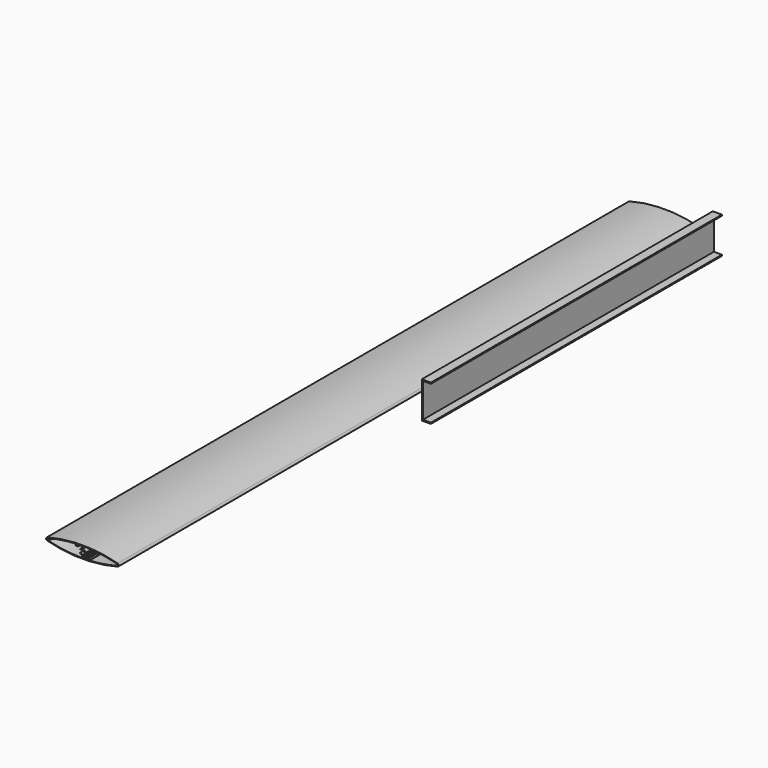
from build123d import *

# Parameters (mm, degrees)
F1_DEPTH = 2000
F3_DEPTH = 1000


# Not quite as in the source:
# - ends of sketch curves that miss each other by under 0.0002 mm in the source are joined


with BuildPart() as f1:
    # F0 (on Front) → F1 (new body)
    with BuildSketch(Plane.XZ):
        with BuildLine():
            ThreePointArc((-17.5657668552, -7.9557874553), (-114.482143, 4.708559), (-211.3985191448, -7.9557874553))
            ThreePointArc((-211.3985191468, -7.9557874481), (-214.482143, -11.966441), (-211.3985191468, -15.9770945519))
            ThreePointArc((-211.3985191448, -15.9770945447), (-114.482143, -28.641441), (-17.5657668552, -15.9770945447))
            ThreePointArc((-17.5657668532, -15.9770945519), (-14.482143, -11.966441), (-17.5657668532, -7.9557874481))
        make_face()
        with BuildLine():
            ThreePointArc((-208.9077742877, -13.5769296747), (-212.482143, -11.966441), (-208.9077742877, -10.3559523253))
            ThreePointArc((-208.9077742877, -10.3559523253), (-207.7533400412, -10.4775188222), (-207.2617892935, -9.425913054))
            ThreePointArc((-207.2617892935, -9.425913054), (-207.1910048941, -9.0656220914), (-206.8932051271, -8.8508305))
            ThreePointArc((-206.8932051271, -8.8508305), (-170.9950203177, -1.5722317693), (-134.5581469899, 2.1710198123))
            ThreePointArc((-134.5581469899, 2.1710198123), (-133.7402264674, 1.8171851888), (-133.5293940092, 0.9513082288))
            ThreePointArc((-133.5293940092, 0.9513082288), (-133.5025335267, -0.9954988279), (-132.5907607495, -2.7158037784))
            ThreePointArc((-132.5907607495, -2.7158037784), (-131.1791989669, -2.8023715374), (-131.0926316821, -1.3908097188))
            ThreePointArc((-131.0926316821, -1.3908097188), (-129.482143, 2.183559), (-127.8716543253, -1.3908097123))
            ThreePointArc((-127.8716543253, -1.3908097123), (-127.7850870331, -2.8023715374), (-126.3735252432, -2.7158037849))
            ThreePointArc((-126.3735252432, -2.7158037849), (-125.4236024617, -0.8328985575), (-125.5217918168, 1.2737680574))
            ThreePointArc((-125.5217918168, 1.2737680574), (-125.3812649978, 2.1537940521), (-124.5944440182, 2.5722506744))
            ThreePointArc((-124.5944440182, 2.5722506744), (-120.5413197711, 2.6596262173), (-116.4874880026, 2.7031994831))
            ThreePointArc((-116.4874880026, 2.7031994831), (-115.776928495, 2.412208007), (-115.482143, 1.703214))
            Line((-115.482143, 1.703214), (-115.482143, -2.986463))
            ThreePointArc((-115.482143, -2.986463), (-115.7019536269, -3.6120063974), (-116.2647520841, -3.9625476222))
            ThreePointArc((-116.2647520841, -3.9625476222), (-118.8659014588, -5.03660249), (-120.9507289205, -6.926858062))
            ThreePointArc((-120.9507289205, -6.926858062), (-120.7764600793, -8.3302931018), (-119.3730248982, -8.1560240793))
            ThreePointArc((-119.3730248982, -8.1560240793), (-108.282143, -11.966441), (-119.3730247168, -15.7768577794))
            ThreePointArc((-119.3730247168, -15.7768577794), (-120.7764600793, -15.6025888982), (-120.9507291018, -17.0060240793))
            ThreePointArc((-120.9507291018, -17.0060240793), (-118.8659014588, -18.89627951), (-116.2647520265, -19.9703341189))
            ThreePointArc((-116.2647520265, -19.9703341189), (-115.7019536269, -20.3208756026), (-115.482143, -20.946419))
            Line((-115.482143, -20.946419), (-115.482143, -25.636096))
            ThreePointArc((-115.482143, -25.636096), (-115.776928495, -26.345090007), (-116.4874880038, -26.6360817154))
            ThreePointArc((-116.4874880038, -26.6360817154), (-162.0425086737, -23.6145958983), (-206.8932050038, -15.0820510151))
            ThreePointArc((-206.8932050038, -15.0820510151), (-207.1910048941, -14.8672599086), (-207.2617897315, -14.5069688654))
            ThreePointArc((-207.2617897315, -14.5069688654), (-207.7533400412, -13.4553631778), (-208.9077742877, -13.5769296747))
        make_face(mode=Mode.SUBTRACT)
        with BuildLine():
            ThreePointArc((-112.6995339159, -3.9625476222), (-113.2623323731, -3.6120063974), (-113.482143, -2.986463))
            Line((-113.482143, -2.986463), (-113.482143, 1.703214))
            ThreePointArc((-113.482143, 1.703214), (-113.187357505, 2.412208007), (-112.4767979962, 2.7031997154))
            ThreePointArc((-112.4767979962, 2.7031997154), (-66.9217773263, -0.3182861017), (-22.0710809962, -8.8508309849))
            ThreePointArc((-22.0710809962, -8.8508309849), (-21.7732811059, -9.0656220914), (-21.7024962685, -9.4259131346))
            ThreePointArc((-21.7024962685, -9.4259131346), (-21.2109459588, -10.4775188222), (-20.0565117188, -10.3559523179))
            ThreePointArc((-20.0565117188, -10.3559523179), (-16.482143, -11.966441), (-20.0565117123, -13.5769296747))
            ThreePointArc((-20.0565117123, -13.5769296747), (-21.2109459588, -13.4553631778), (-21.7024967065, -14.506968946))
            ThreePointArc((-21.7024967065, -14.506968946), (-21.7732811059, -14.8672599086), (-22.0710808729, -15.0820515))
            ThreePointArc((-22.0710808729, -15.0820515), (-57.9692656823, -22.3606502307), (-94.4061390101, -26.1039018123))
            ThreePointArc((-94.4061390101, -26.1039018123), (-95.2240595326, -25.7500671888), (-95.4348919908, -24.8841902288))
            ThreePointArc((-95.4348919908, -24.8841902288), (-95.4617524733, -22.9373831721), (-96.3735252505, -21.2170782216))
            ThreePointArc((-96.3735252505, -21.2170782216), (-97.7850870331, -21.1305104626), (-97.8716543179, -22.5420722812))
            ThreePointArc((-97.8716543179, -22.5420722812), (-99.482143, -26.116441), (-101.0926316747, -22.5420722877))
            ThreePointArc((-101.0926316747, -22.5420722877), (-101.1791989669, -21.1305104626), (-102.5907607568, -21.2170782151))
            ThreePointArc((-102.5907607568, -21.2170782151), (-103.5406835383, -23.0999834425), (-103.4424941832, -25.2066500574))
            ThreePointArc((-103.4424941832, -25.2066500574), (-103.5830210022, -26.0866760521), (-104.3698419818, -26.5051326744))
            ThreePointArc((-104.3698419818, -26.5051326744), (-108.4229662289, -26.5925082173), (-112.4767979974, -26.6360814831))
            ThreePointArc((-112.4767979974, -26.6360814831), (-113.187357505, -26.345090007), (-113.482143, -25.636096))
            Line((-113.482143, -25.636096), (-113.482143, -20.946419))
            ThreePointArc((-113.482143, -20.946419), (-113.2623323731, -20.3208756026), (-112.6995339159, -19.9703343778))
            ThreePointArc((-112.6995339159, -19.9703343778), (-108.2086364539, -17.2468875357), (-106.291455428, -12.3571289796))
            Line((-106.291455428, -12.3571289796), (-106.682143, -11.966441))
            Line((-106.682143, -11.966441), (-106.291455, -11.575753))
            ThreePointArc((-106.291455, -11.575753), (-108.2086364539, -6.6859944643), (-112.6995339159, -3.9625476222))
        make_face(mode=Mode.SUBTRACT)
    extrude(amount=F1_DEPTH)


with BuildPart() as f3:
    # F2 (on Front) → F3 (new body)
    with BuildSketch(Plane.XZ):
        Polygon((43.0757822734, 42.6162129075), (18.084763796, 42.6162129075), (18.084763796, -57.3837870925), (43.0757822734, -57.3837870925), (43.084763796, -57.3837870925), (43.0757822733, -54.3838005361), (21.0847503524, -54.3838005361), (21.0847503524, 39.6162263511), (43.0757826234, 39.6162263511), (43.084763796, 42.6162129075), align=None)
    extrude(amount=F3_DEPTH)


solid = Compound([f1.part, f3.part])
